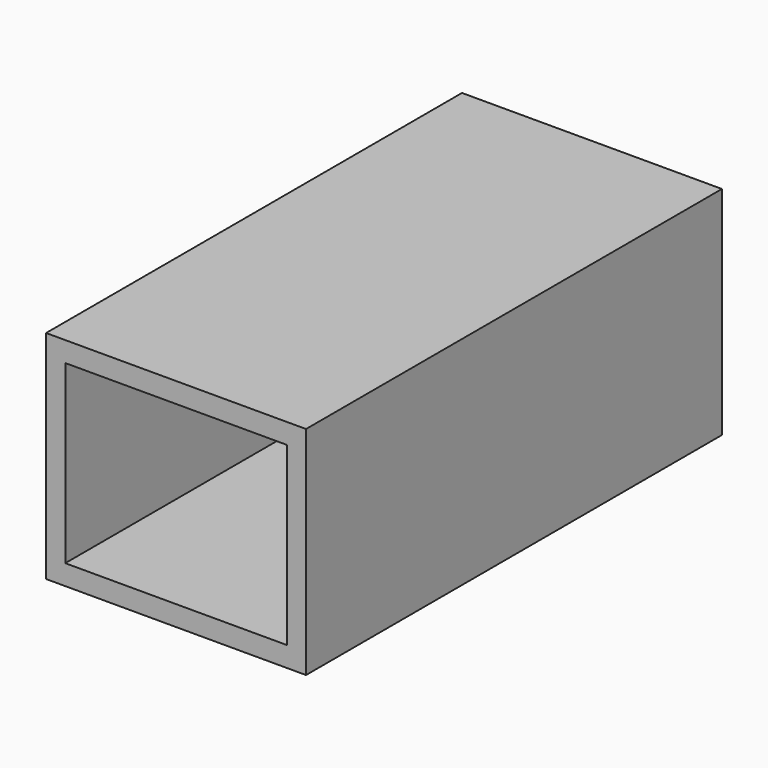
from build123d import *

# Parameters (mm, degrees)
F0_W     = 304.8
F0_H     = 254
F0_W_2   = 259.7959858463
F0_H_2   = 206.6094064729
F1_DEPTH = 609.6


# Not quite as in the source:
# - the program builds the solid bodies; features that only make, move or delete a surface that nothing else refers to are left out


with BuildPart() as f1:
    # F0 (on Front) → F1 (new body)
    with BuildSketch(Plane.XZ):
        Rectangle(F0_W, F0_H)
        Rectangle(F0_W_2, F0_H_2, mode=Mode.SUBTRACT)
    extrude(amount=F1_DEPTH)


solid = f1.part
